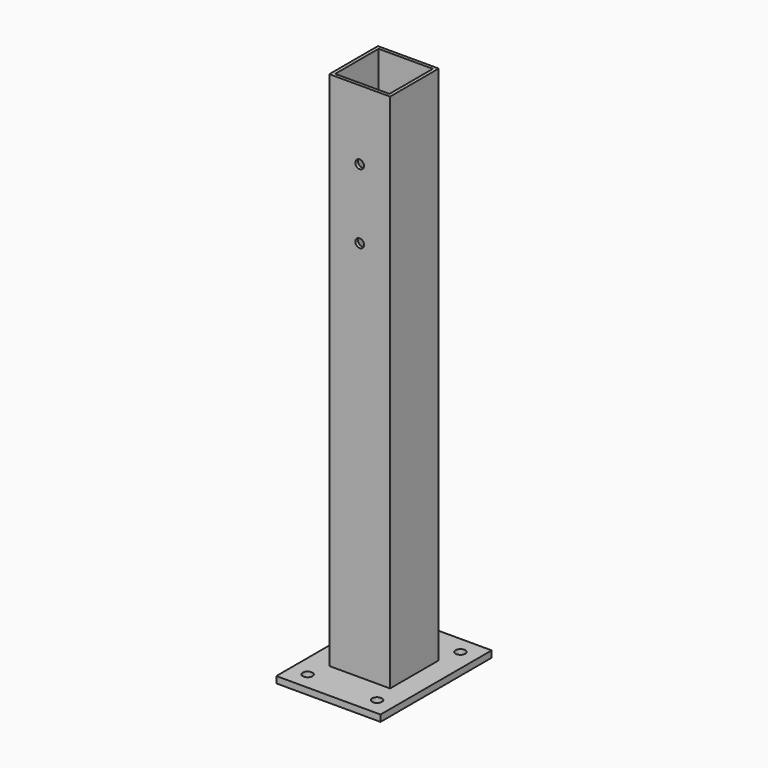
from build123d import *

# Parameters (mm, degrees)
F0_W        = 152.4
F0_H        = 203.2
F1_DEPTH    = 9.525
F2_W        = 88.9
F2_H        = 88.9
F3_DEPTH    = 762
F4_R        = 7.14375
F5_DEPTH    = 25.4
F7_T        = 4.7625
F7_T3_DEPTH = 98.425
F7_T5_DEPTH = 98.425
F6_R        = 6.35
F8_DEPTH    = 25.4


# Not quite as in the source:
# - a shell that OpenCascade refuses in one call is made with other operations: the cavity is built on its own and cut out


with BuildPart() as f1:
    # F0 (on Top) → F1 (new body)
    with BuildSketch(Plane.XY):
        with Locations((76.2, 101.6)):
            Rectangle(F0_W, F0_H)
    extrude(amount=F1_DEPTH)

    # F2 (on face) → F3 (join)
    with BuildSketch(Plane.XY.offset(9.525)):
        with Locations((76.2, 101.6)):
            Rectangle(F2_W, F2_H)
    extrude(amount=F3_DEPTH)

    # F4 (on face) → F5 (cut)
    with BuildSketch(Plane.XY.offset(9.525)):
        with Locations((127, 177.8)):
            Circle(F4_R)
        with Locations((127, 25.4)):
            Circle(F4_R)
        with Locations((25.4, 25.4)):
            Circle(F4_R)
        with Locations((25.4, 177.8)):
            Circle(F4_R)
    extrude(amount=-F5_DEPTH, mode=Mode.SUBTRACT)

    # F7: shell of thickness 4.7625, made by hand


with BuildPart() as f7_core1:
    # F7_t2: copy of F1
    add(f1.part)

    # the walls: a layer under each face that stays
    f7_faces = [f7_core1.faces().sort_by_distance(p)[0] for p in [
        (0, 101.6, 4.7625),
        (76.2, 203.2, 4.7625),
        (76.2, 0, 4.7625),
        (76.2, 101.6, 0),
        (25.4, 33.8666666667, 9.525),
        (152.4, 101.6, 4.7625),
        (18.25625, 25.4, 4.7625),
        (119.85625, 25.4, 4.7625),
        (18.25625, 177.8, 4.7625),
        (119.85625, 177.8, 4.7625),
        (120.65, 101.6, 390.525),
        (76.2, 57.15, 390.525),
        (76.2, 146.05, 390.525),
        (31.75, 101.6, 390.525),
    ]]
    thicken(f7_faces, amount=-F7_T, mode=Mode.SUBTRACT)

    # F7_s4 → F7_t3 (cut)
    with BuildSketch(Plane.XZ.offset(-150.8125)):
        Polygon((120.697625, 9.572625), (120.65, 4.7625), (115.8875, 4.7625), (115.8875, 9.525), align=None)
        Polygon((31.702375, 9.572625), (31.75, 4.7625), (36.5125, 4.7625), (36.5125, 9.525), align=None)
    extrude(amount=F7_T3_DEPTH, mode=Mode.SUBTRACT)

    # F7_s6 → F7_t5 (cut)
    with BuildSketch(Plane.YZ.offset(26.9875)):
        Polygon((57.102375, 9.572625), (57.15, 4.7625), (61.9125, 4.7625), (61.9125, 9.525), align=None)
        Polygon((146.097625, 9.572625), (146.05, 4.7625), (141.2875, 4.7625), (141.2875, 9.525), align=None)
    extrude(amount=F7_T5_DEPTH, mode=Mode.SUBTRACT)


with BuildPart() as f1_1:
    add(f1.part)

    # what is left inside the walls is the cavity
    f7_cavity = [f7_core1.part.solids().sort_by_distance(p)[0] for p in [
        (36.560125, 88.370833, 388.14375),
    ]]
    add(f7_cavity, mode=Mode.SUBTRACT)

    # F6 (on face) → F8 (cut)
    with BuildSketch(Plane.XZ.offset(-57.15)):
        with Locations((76.2, 669.925)):
            Circle(F6_R)
        with Locations((76.2, 568.325)):
            Circle(F6_R)
    extrude(amount=-F8_DEPTH, mode=Mode.SUBTRACT)


solid = f1_1.part
